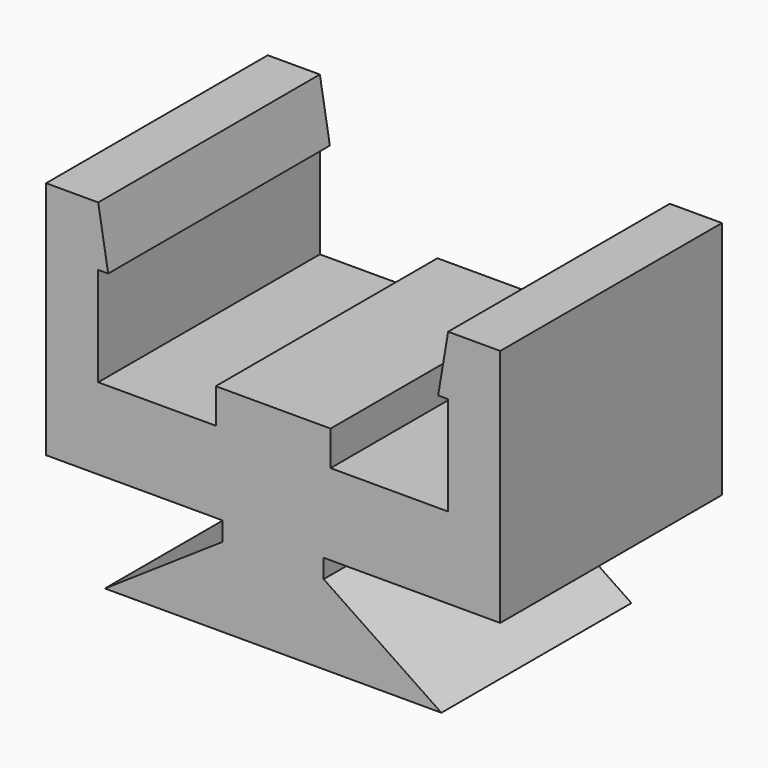
from build123d import *

# Parameters (mm, degrees)
F1_DEPTH = 7
F3_DEPTH = 1


# Not quite as in the source:
# - ends of sketch curves that miss each other by under 0.0002 mm in the source are joined


with BuildPart() as f1:
    # F0 (on Front) → F1 (new body)
    with BuildSketch(Plane.XZ):
        Polygon((-1.4500004135, 5.0060716327), (-2.9995756401, 5.0060716327), (-4.4200004135, 5.0060716327), (-4.4200004135, 7.5060716327), (-4.1678175591, 7.5060716327), (-4.4200004135, 9.0056643691), (-5.7365144081, 9.0056643691), (-5.7365144081, 2.9560173731), (-1.276, 2.9560173731), (-1.276, 2.479687877), (-4.25, 0.475687877), (0, 0.475687877), (4.25, 0.475687877), (1.276, 2.479687877), (1.276, 2.9560173731), (5.7365144081, 2.9560173731), (5.7365144081, 9.0056643691), (4.4200002068, 9.0056643691), (4.1678173524, 7.5060716327), (4.4200002068, 7.5060716327), (4.4200002068, 5.0060716327), (2.9995754333, 5.0060716327), (1.4500002068, 5.0060716327), (2.068e-07, 5.0060716327), align=None)
        Polygon((-1.4500004135, 5.8852624949), (-1.4500004135, 5.0060716327), (-4.135e-07, 5.0060716327), (1.4500002068, 5.0060716327), (1.4500002068, 5.8852624949), (2.068e-07, 5.8852624949), align=None)
    extrude(amount=F1_DEPTH)

    # F2 (on face) → F3 (cut)
    with BuildSketch(Plane(origin=(0, 0, 0), x_dir=(-1, 0, 0), z_dir=(0, 1, 0))):
        Polygon((1.276, 2.9560173731), (-1.276, 2.9560173731), (-1.276, 2.479687877), (-4.25, 0.475687877), (4.25, 0.475687877), (1.276, 2.479687877), align=None)
    extrude(amount=-F3_DEPTH, mode=Mode.SUBTRACT)


solid = f1.part
